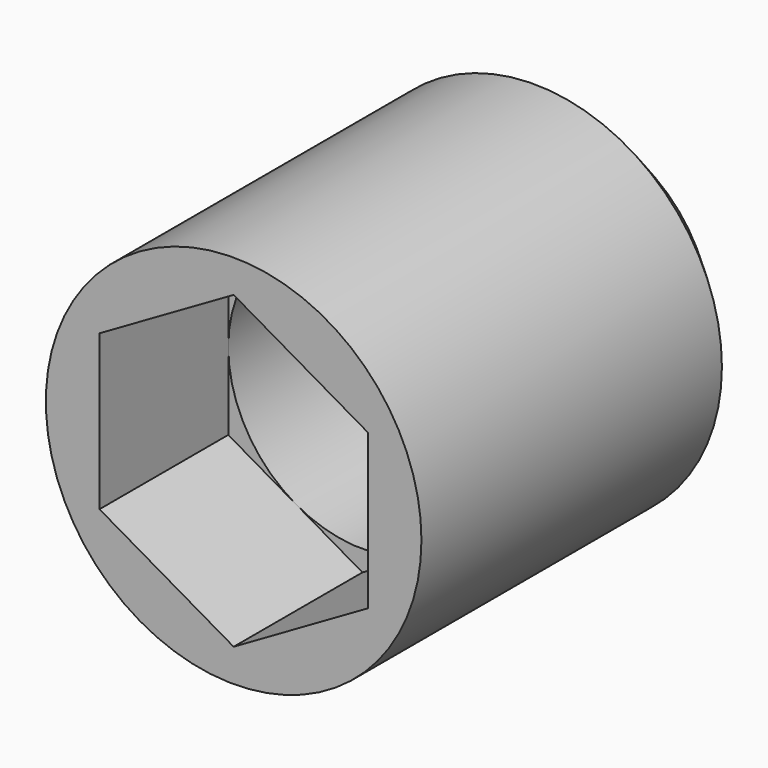
from build123d import *

# Parameters (mm, degrees)
F0_R     = 3.5
F1_DEPTH = 8
F3_DEPTH = 3
F4_R     = 2.5
F5_DEPTH = 25
F6_SIZE  = 0.99999


# Not quite as in the source:
# - a fillet or chamfer is up to 0.001 mm smaller than in the source, because OpenCascade refuses the exact size


with BuildPart() as f1:
    # F0 (on Front) → F1 (new body)
    with BuildSketch(Plane.XZ):
        Circle(F0_R)
    extrude(amount=F1_DEPTH)

    # F2 (on face) → F3 (cut)
    with BuildSketch(Plane.XZ.offset(8)):
        Polygon((2.5, 1.443375673), (0, 2.8867513459), (-2.5, 1.443375673), (-2.5, -1.443375673), (0, -2.8867513459), (2.5, -1.443375673), align=None)
    extrude(amount=-F3_DEPTH, mode=Mode.SUBTRACT)

    # F4 (on face) → F5 (cut)
    with BuildSketch(Plane.XZ.offset(5)):
        Circle(F4_R)
    extrude(amount=-F5_DEPTH, mode=Mode.SUBTRACT)

    # F6 (size 1 in the source; OpenCascade refuses exactly that, so slightly less here)
    f6_edges = [f1.edges().sort_by_distance(p)[0] for p in [
        (-3.5, 0, 0),
    ]]
    chamfer(f6_edges, length=F6_SIZE)


solid = f1.part
